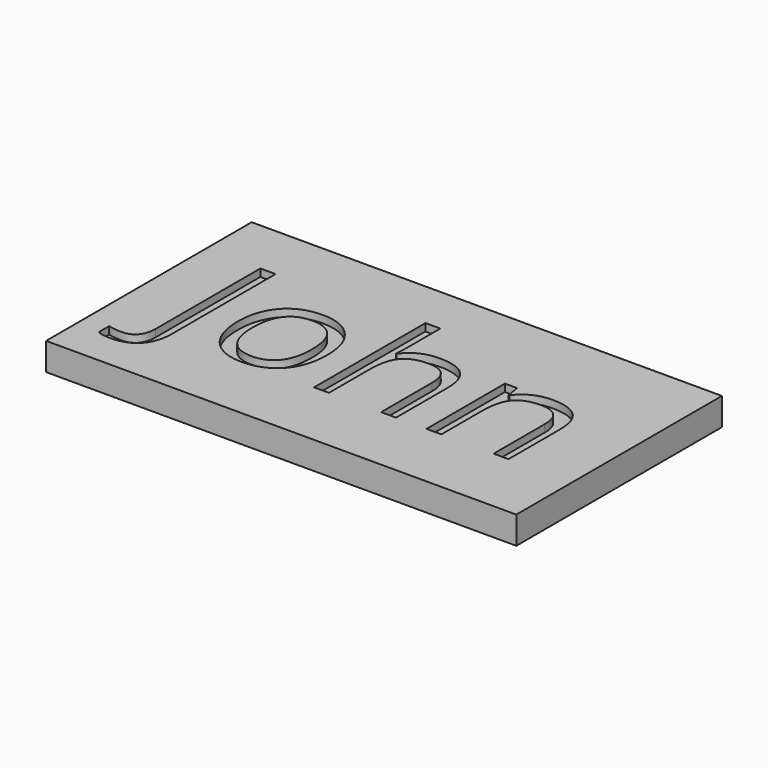
from build123d import *

# Parameters (mm, degrees)
F1_DEPTH     = 9.398
F2_TEXT_SIZE = 62.6168369594
F3_DEPTH     = 2.54


# Not quite as in the source:
# - Text() gives the source's letters only with a copy of the font that has no kerning and outlines rounded to 1/6400 em; it was checked with that copy


with BuildPart() as f1:
    # F0 (on Top) → F1 (new body)
    with BuildSketch(Plane.XY):
        Polygon((25.3923758864, 47.0562539995), (-71.9859004021, 47.0562539995), (-71.9859004021, -34.5715545118), (-71.9859004021, -40.7814793289), (88.7349545956, -40.7814793289), (88.7349545956, 47.0562539995), align=None)
    extrude(amount=F1_DEPTH)

    # F2 (on face) → F3 (cut)
    with BuildSketch(Plane.XY.offset(9.398)):
        with Locations((-59.2859004021, -17.0778686113)):
            Text('John', F2_TEXT_SIZE, font='Open Sans', text_align=(TextAlign.LEFT, TextAlign.BOTTOM))
    extrude(amount=-F3_DEPTH, mode=Mode.SUBTRACT)


solid = f1.part
